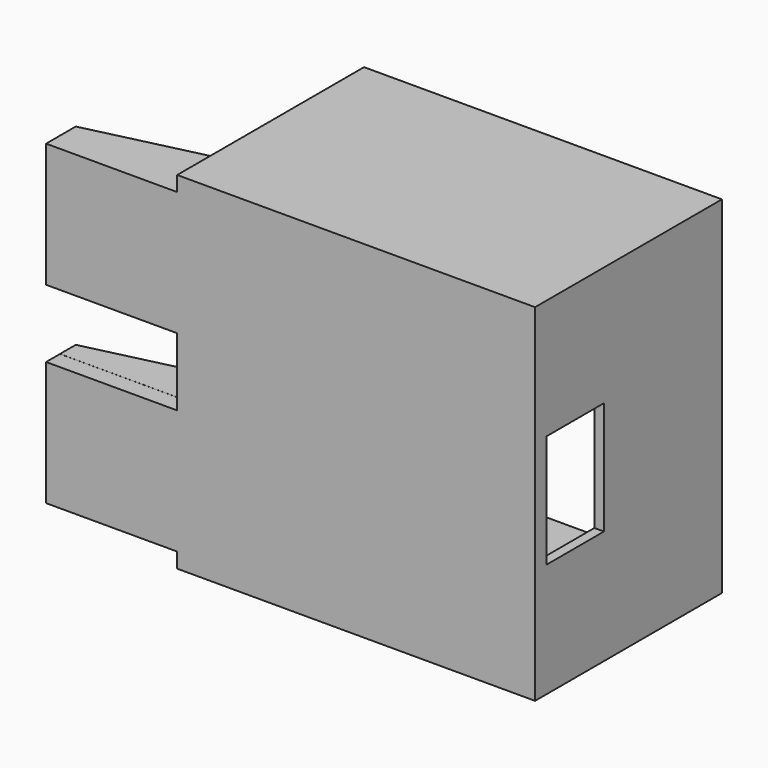
from build123d import *

# Parameters (mm, degrees)
F0_W      = 475
F0_H      = 310
F1_DEPTH  = 115
F2_T      = -12.7
F3_W      = 93
F3_H      = 125
F3_H_2    = 135
F4_DEPTH  = 25
F5_DEPTH  = 25
F7_DEPTH  = 174
F8_W      = 15
F8_H      = 125
F10_DEPTH = 35
F11_DEPTH = 363
F13_W     = 42.5
F13_H     = 7.8922572035
F13_W_2   = 40
F13_H_2   = 48.3056434989
F13_H_3   = 48.6943565011
F13_H_4   = 8.1077427965
F14_DEPTH = 25
F15_W     = 95
F15_H     = 150
F16_DEPTH = 25
F13_R     = 15.5
F17_DEPTH = 25


# Not quite as in the source:
# - a feature names something its author has since deleted; it is built from what else it names


with BuildPart() as f1:
    # F0 (on Top) → F1 (new body, symmetric)
    with BuildSketch(Plane.XY):
        Rectangle(F0_W, F0_H)
    extrude(amount=F1_DEPTH, both=True)

    # F2
    f2_openings = [f1.faces().sort_by_distance(p)[0] for p in [
        (0, 0, 115),
    ]]
    offset(amount=F2_T, openings=f2_openings)

    # F3 (on face) → F4 (cut)
    with BuildSketch(Plane(origin=(-237.5, 0, 0), x_dir=(0, -1, 0), z_dir=(-1, 0, 0))):
        with Locations((85.4776808544, -12.5305280089)):
            Rectangle(F3_W, F3_H)
        with Locations((-50.0830374043, -7.5305280089)):
            Rectangle(F3_W, F3_H_2)
    extrude(amount=-F4_DEPTH, mode=Mode.SUBTRACT)

    # F5 (cut): a face of the model
    f5_faces = [f1.faces().sort_by_distance(p)[0] for p in [
        (0, 142.3, 6.35),
    ]]
    extrude(f5_faces, amount=-F5_DEPTH, mode=Mode.SUBTRACT)

    # F6 (on face) → F7 (join)
    with BuildSketch(Plane(origin=(-237.5, 0, 0), x_dir=(0, -1, 0), z_dir=(-1, 0, 0))):
        Polygon((131.9776808544, -75.0305280089), (38.9776808544, -75.0305280089), (38.9776808544, -95.0305280089), (131.9776808544, -95.0305280089), (155, -95.0305280089), (155, 69.9025020003), (131.9776808544, 69.9025020003), (131.9776808544, 69.9694719911), (38.9776808544, 69.9694719911), (38.9776808544, 49.9694719911), (131.9776808544, 49.9694719911), align=None)
    extrude(amount=F7_DEPTH)

    # F8 (on face) → F10 (join)
    with BuildSketch(Plane(origin=(0, -131.9776808544, 0), x_dir=(-1, 0, 0), z_dir=(0, 1, 0))):
        with Locations((404, -12.5305280089)):
            Rectangle(F8_W, F8_H)
    extrude(amount=F10_DEPTH)

    # F9 (on face) → F11 (cut)
    with BuildSketch(Plane(origin=(0, 0, -95.0305280089), x_dir=(1, 0, 0), z_dir=(0, 0, -1))):
        Polygon((-411.5, 38.9776808544), (-237.5, 38.9776808544), (-237.5, 64.5424127579), (-411.5, 105.7684645057), align=None)
    extrude(amount=-F11_DEPTH, mode=Mode.SUBTRACT)

    # F12: F1 across face


with BuildPart() as f1_1:
    add(f1.part)
    add(f1.part.mirror(Plane(origin=(0, -62.4841436051, 115), x_dir=(1, 0, 0), z_dir=(0, 0, 1))))

    # F13 (on face) → F14 (cut)
    with BuildSketch(Plane(origin=(-237.5, 0, 0), x_dir=(0, -1, 0), z_dir=(-1, 0, 0))):
        with Locations((85.7924127579, 118.9461286017)):
            Rectangle(F13_W, F13_H)
        with Locations((-23.5830374043, 90.8471782506)):
            Rectangle(F13_W_2, F13_H_2)
        with Locations((-23.5830374043, 139.3471782506)):
            Rectangle(F13_W_2, F13_H_3)
        with Locations((85.7924127579, 110.9461286017)):
            Rectangle(F13_W, F13_H_4)
    extrude(amount=-F14_DEPTH, mode=Mode.SUBTRACT)

    # F15 (on face) → F16 (cut)
    with BuildSketch(Plane.YZ.offset(237.5)):
        with Locations((-88.2316343486, 111.4078534107)):
            Rectangle(F15_W, F15_H)
    extrude(amount=-F16_DEPTH, mode=Mode.SUBTRACT)

    # F13 (on face) → F17 (cut)
    with BuildSketch(Plane(origin=(-237.5, 0, 0), x_dir=(0, -1, 0), z_dir=(-1, 0, 0))):
        with Locations((17.697321725, 166.6680857539)):
            Circle(F13_R)
        with BuildLine():
            ThreePointArc((33.197321725, 63.3319142461), (17.697321725, 78.8319142461), (2.197321725, 63.3319142461))
            Line((2.197321725, 63.3319142461), (17.697321725, 63.3319142461))
            Line((17.697321725, 63.3319142461), (33.197321725, 63.3319142461))
        make_face()
        with BuildLine():
            Line((17.697321725, 63.3319142461), (2.197321725, 63.3319142461))
            ThreePointArc((2.197321725, 63.3319142461), (17.697321725, 47.8319142461), (33.197321725, 63.3319142461))
            Line((33.197321725, 63.3319142461), (17.697321725, 63.3319142461))
        make_face()
    extrude(amount=-F17_DEPTH, mode=Mode.SUBTRACT)


solid = f1_1.part
